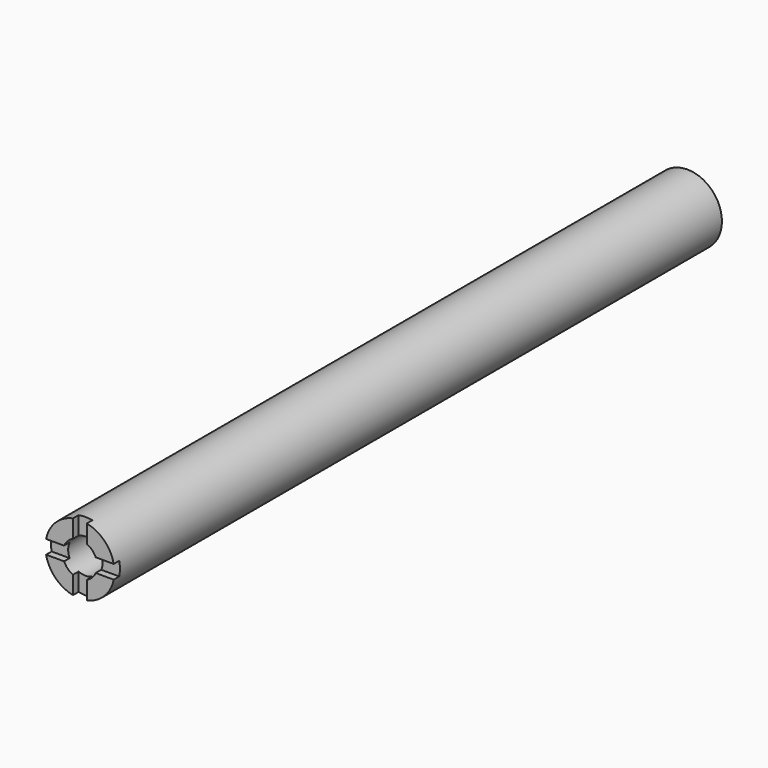
from build123d import *

# Parameters (mm, degrees)
F0_R     = 12.7
F0_R_2   = 6.35
F1_DEPTH = 279.4
F3_DEPTH = 2.54


with BuildPart() as f1:
    # F0 (on Front) → F1 (new body)
    with BuildSketch(Plane.XZ):
        Circle(F0_R)
        Circle(F0_R_2, mode=Mode.SUBTRACT)
    extrude(amount=F1_DEPTH)

    # F2 (on face) → F3 (cut)
    with BuildSketch(Plane.XZ.offset(279.4)):
        with BuildLine():
            Line((2.54, 5.8198711326), (2.54, 12.4434078933))
            ThreePointArc((2.54, 12.4434078933), (0, 12.7), (-2.54, 12.4434078933))
            Line((-2.54, 12.4434078933), (-2.54, 5.8198711326))
            ThreePointArc((-2.54, 5.8198711326), (0, 6.35), (2.54, 5.8198711326))
        make_face()
        with BuildLine():
            Line((-5.8198711326, 2.54), (-12.4434078933, 2.54))
            ThreePointArc((-12.4434078933, 2.54), (-12.7, 0), (-12.4434078933, -2.54))
            Line((-12.4434078933, -2.54), (-5.8198711326, -2.54))
            ThreePointArc((-5.8198711326, -2.54), (-6.35, 0), (-5.8198711326, 2.54))
        make_face()
        with BuildLine():
            ThreePointArc((-2.54, -12.4434078933), (0, -12.7), (2.54, -12.4434078933))
            Line((2.54, -12.4434078933), (2.54, -5.8198711326))
            ThreePointArc((2.54, -5.8198711326), (0, -6.35), (-2.54, -5.8198711326))
            Line((-2.54, -5.8198711326), (-2.54, -12.4434078933))
        make_face()
        with BuildLine():
            ThreePointArc((12.4434078933, -2.54), (12.6356891432, -1.2764638175), (12.7, 0))
            ThreePointArc((12.7, 0), (12.6356891432, 1.2764638175), (12.4434078933, 2.54))
            Line((12.4434078933, 2.54), (5.8198711326, 2.54))
            ThreePointArc((5.8198711326, 2.54), (6.2160550871, 1.2973662374), (6.35, 0))
            ThreePointArc((6.35, 0), (6.2160550871, -1.2973662374), (5.8198711326, -2.54))
            Line((5.8198711326, -2.54), (12.4434078933, -2.54))
        make_face()
    extrude(amount=-F3_DEPTH, mode=Mode.SUBTRACT)


solid = f1.part
